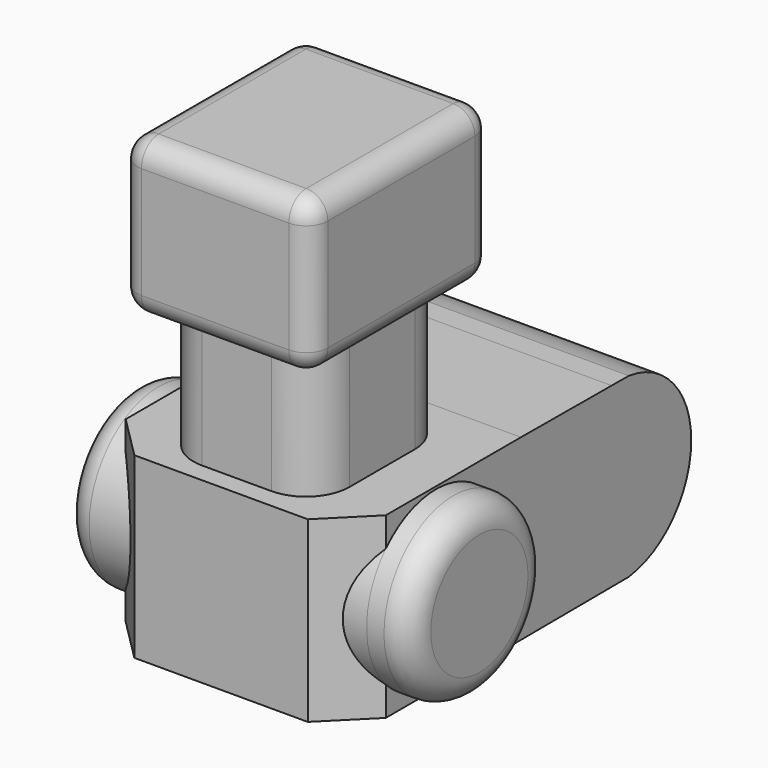
from build123d import *

# Parameters (mm, degrees)
F0_W          = 194.5625826716
F0_H          = 54.5296296477
F1_DEPTH      = 90
F0_W_2        = 261.9621157646
F0_H_2        = 41.3846671581
F0_H_3        = 48.0061769485
F2_DEPTH      = 110
F3_DEPTH      = 150
F4_DEPTH      = 200
F5_T1_DEPTH   = 170
F5_T3_DEPTH   = 211.9621157646
F5_T5_DEPTH   = 128.7816882133
F5_S9_W       = 25
F5_S9_H       = 25
F5_T10_DEPTH  = 25
F5_S15_W      = 25
F5_S15_H      = 25
F5_T16_DEPTH  = 25
F5_S21_W      = 25
F5_S21_H      = 25
F5_T22_DEPTH  = 25
F5_S27_W      = 25
F5_S27_H      = 25
F5_T28_DEPTH  = 25
F5_S33_W      = 25
F5_S33_H      = 25
F5_T34_DEPTH  = 25
F5_S39_W      = 25
F5_S39_H      = 25
F5_T40_DEPTH  = 25
F5_S45_W      = 25
F5_S45_H      = 25
F5_T46_DEPTH  = 25
F5_S51_W      = 25
F5_S51_H      = 25
F5_T52_DEPTH  = 25
F5_T58_DEPTH  = 211.9621157646
F5_T64_DEPTH  = 211.9621157646
F5_T70_DEPTH  = 211.9621157646
F5_T77_DEPTH  = 211.9621157646
F5_T83_DEPTH  = 211.9621157646
F5_T89_DEPTH  = 211.9621157646
F5_T95_DEPTH  = 211.9621157646
F5_T101_DEPTH = 211.9621157646
F5_T108_DEPTH = 211.9621157646
F5_T114_DEPTH = 211.9621157646
F6_R          = 50
F8_T4_DEPTH   = 462.9335014381
F8_S5_R       = 100
F8_T6_DEPTH   = 236
F8_T10_DEPTH  = 462.9335014381
F8_S11_R      = 100
F8_T12_DEPTH  = 236


# Not quite as in the source:
# - a fillet or chamfer that OpenCascade refuses, or shapes differently, is made with other operations: its cross-section is extruded or revolved along the edge and cut away or added


with BuildPart() as f1:
    # F0 (on Right) → F1 (new body, symmetric)
    with BuildSketch(Plane.YZ):
        with Locations((-2.7187086642, 130.1474161446)):
            Rectangle(F0_W, F0_H)
        Polygon((-100, 210.3845775127), (-100, 157.4122309685), (94.5625826716, 157.4122309685), (94.5625826716, 209.366121575), align=None)
        Polygon((-100, 248.4584450722), (-100, 210.3845775127), (94.5625826716, 209.366121575), (94.5625826716, 248.4584450722), align=None)
    extrude(amount=F1_DEPTH, both=True)

    # F0 (on Right) → F2 (join, symmetric)
    with BuildSketch(Plane.YZ):
        Polygon((-130.9810578823, 248.4584450722), (-100, 248.4584450722), (94.5625826716, 248.4584450722), (130.9810578823, 248.4584450722), (130.9810578823, 296.4646220207), (-130.9810578823, 296.4646220207), align=None)
        with Locations((0, 317.1569555998)):
            Rectangle(F0_W_2, F0_H_2)
        with Locations((0, 361.8523776531)):
            Rectangle(F0_W_2, F0_H_3)
        with Locations((0, 406.5477997065)):
            Rectangle(F0_W_2, F0_H_2)
    extrude(amount=F2_DEPTH, both=True)

    # F0 (on Right) → F3 (join, symmetric)
    with BuildSketch(Plane.YZ):
        with BuildLine():
            ThreePointArc((100, 0), (0, -100), (-100, 0))
            Line((-100, 0), (-100, 102.8826013207))
            Line((-100, 102.8826013207), (-122.4384903908, 102.8826013207))
            Line((-122.4384903908, 102.8826013207), (-122.4384903908, -102.8826013207))
            Line((-122.4384903908, -102.8826013207), (122.4384903908, -102.8826013207))
            Line((122.4384903908, -102.8826013207), (122.4384903908, 102.8826013207))
            Line((122.4384903908, 102.8826013207), (94.5625826716, 102.8826013207))
            Line((94.5625826716, 102.8826013207), (94.5625826716, 32.525650777))
            ThreePointArc((94.5625826716, 32.525650777), (98.6312786776, 16.4885071009), (100, 0))
        make_face()
        with BuildLine():
            Line((253.218506448, 102.1980211612), (122.4384903908, 102.8826013207))
            Line((122.4384903908, 102.8826013207), (122.4384903908, -102.8826013207))
            Line((122.4384903908, -102.8826013207), (253.218506448, -102.1980211612))
            ThreePointArc((253.218506448, -102.1980211612), (162.1847078204, 0), (253.218506448, 102.1980211612))
        make_face()
        with BuildLine():
            Line((277.9853632955, 102.0683767451), (253.218506448, 102.1980211612))
            ThreePointArc((253.218506448, 102.1980211612), (162.1847078204, 0), (253.218506448, -102.1980211612))
            Line((253.218506448, -102.1980211612), (277.9853632955, -102.0683767451))
            Line((277.9853632955, -102.0683767451), (277.9853632955, 102.0683767451))
        make_face()
        with BuildLine():
            ThreePointArc((367.9499104619, 0), (342.2485007293, 68.0286213263), (277.9853632955, 102.0683767451))
            Line((277.9853632955, 102.0683767451), (277.9853632955, -102.0683767451))
            ThreePointArc((277.9853632955, -102.0683767451), (342.2485007293, -68.0286213263), (367.9499104619, 0))
        make_face()
        with BuildLine():
            Line((-100, 102.8826013207), (-100, 0))
            ThreePointArc((-100, 0), (-16.4885071009, 98.6312786776), (94.5625826716, 32.525650777))
            Line((94.5625826716, 32.525650777), (94.5625826716, 102.8826013207))
            Line((94.5625826716, 102.8826013207), (-100, 102.8826013207))
        make_face()
    extrude(amount=F3_DEPTH, both=True)

    # F0 (on Right) → F4 (join, symmetric)
    with BuildSketch(Plane.YZ):
        with BuildLine():
            ThreePointArc((94.5625826716, 32.525650777), (-16.4885071009, 98.6312786776), (-100, 0))
            Line((-100, 0), (94.5625826716, 0))
            Line((94.5625826716, 0), (94.5625826716, 32.525650777))
        make_face()
        with BuildLine():
            Line((94.5625826716, 0), (-100, 0))
            ThreePointArc((-100, 0), (0, -100), (100, 0))
            ThreePointArc((100, 0), (98.6312786776, 16.4885071009), (94.5625826716, 32.525650777))
            Line((94.5625826716, 32.525650777), (94.5625826716, 0))
        make_face()
    extrude(amount=F4_DEPTH, both=True)

    # F5: fillet of radius 25 on 12 edges, made by hand

    # F5_s2 → F5_t1 (cut)
    with BuildSketch(Plane.YZ.offset(-85)):
        with BuildLine():
            ThreePointArc((-130.9810578823, 402.2401332855), (-123.658727412, 419.9178028152), (-105.9810578823, 427.2401332855))
            Line((-105.9810578823, 427.2401332855), (-130.9810578823, 427.2401332855))
            Line((-130.9810578823, 427.2401332855), (-130.9810578823, 402.2401332855))
        make_face()
        with BuildLine():
            ThreePointArc((130.9810578823, 402.2401332855), (123.658727412, 419.9178028152), (105.9810578823, 427.2401332855))
            Line((105.9810578823, 427.2401332855), (130.9810578823, 427.2401332855))
            Line((130.9810578823, 427.2401332855), (130.9810578823, 402.2401332855))
        make_face()
        with BuildLine():
            ThreePointArc((-105.9810578823, 248.4584450722), (-123.658727412, 255.7807755425), (-130.9810578823, 273.4584450722))
            Line((-130.9810578823, 273.4584450722), (-130.9810578823, 248.4584450722))
            Line((-130.9810578823, 248.4584450722), (-105.9810578823, 248.4584450722))
        make_face()
        with BuildLine():
            ThreePointArc((105.9810578823, 248.4584450722), (123.658727412, 255.7807755425), (130.9810578823, 273.4584450722))
            Line((130.9810578823, 273.4584450722), (130.9810578823, 248.4584450722))
            Line((130.9810578823, 248.4584450722), (105.9810578823, 248.4584450722))
        make_face()
    extrude(amount=F5_T1_DEPTH, mode=Mode.SUBTRACT)

    # F5_s4 → F5_t3 (cut)
    with BuildSketch(Plane.XZ.offset(-105.9810578823)):
        with BuildLine():
            ThreePointArc((110, 402.2401332855), (102.6776695297, 419.9178028152), (85, 427.2401332855))
            Line((85, 427.2401332855), (110, 427.2401332855))
            Line((110, 427.2401332855), (110, 402.2401332855))
        make_face()
        with BuildLine():
            ThreePointArc((-110, 402.2401332855), (-102.6776695297, 419.9178028152), (-85, 427.2401332855))
            Line((-85, 427.2401332855), (-110, 427.2401332855))
            Line((-110, 427.2401332855), (-110, 402.2401332855))
        make_face()
    extrude(amount=F5_T3_DEPTH, mode=Mode.SUBTRACT)

    # F5_s6 → F5_t5 (cut)
    with BuildSketch(Plane.XY.offset(273.4584450722)):
        with BuildLine():
            ThreePointArc((85, -130.9810578823), (102.6776695297, -123.658727412), (110, -105.9810578823))
            Line((110, -105.9810578823), (110, -130.9810578823))
            Line((110, -130.9810578823), (85, -130.9810578823))
        make_face()
        with BuildLine():
            ThreePointArc((85, 130.9810578823), (102.6776695297, 123.658727412), (110, 105.9810578823))
            Line((110, 105.9810578823), (110, 130.9810578823))
            Line((110, 130.9810578823), (85, 130.9810578823))
        make_face()
        with BuildLine():
            ThreePointArc((-110, -105.9810578823), (-102.6776695297, -123.658727412), (-85, -130.9810578823))
            Line((-85, -130.9810578823), (-110, -130.9810578823))
            Line((-110, -130.9810578823), (-110, -105.9810578823))
        make_face()
        with BuildLine():
            ThreePointArc((-110, 105.9810578823), (-102.6776695297, 123.658727412), (-85, 130.9810578823))
            Line((-85, 130.9810578823), (-110, 130.9810578823))
            Line((-110, 130.9810578823), (-110, 105.9810578823))
        make_face()
    extrude(amount=F5_T5_DEPTH, mode=Mode.SUBTRACT)


with BuildPart() as f5_tool8:
    # F5_s9 → F5_t10 (new body)
    with BuildSketch(Plane.XZ.offset(105.9810578823)):
        with Locations((97.5, 414.7401332855)):
            Rectangle(F5_S9_W, F5_S9_H)
    extrude(amount=F5_T10_DEPTH)

    # F5_s11 → F5_t12 (revolve, cut)
    with BuildSketch(Plane(origin=(85, -105.9810578823, 402.2401332855), x_dir=(-0.7071067812, 0, -0.7071067812), z_dir=(-0.7071067812, 0, 0.7071067812))):
        with BuildLine():
            ThreePointArc((0, -25), (25, 0), (0, 25))
            Line((0, 25), (0, -25))
        make_face()
    revolve(axis=Axis((85, -105.9810578823, 402.2401332855), (0, -1, 0)), mode=Mode.SUBTRACT)


with BuildPart() as f1_1:
    add(f1.part)

    # F5_t7: cut F5_tool8
    add(f5_tool8.part, mode=Mode.SUBTRACT)


with BuildPart() as f5_tool14:
    # F5_s15 → F5_t16 (new body)
    with BuildSketch(Plane.YZ.offset(-85)):
        with Locations((-118.4810578823, 414.7401332855)):
            Rectangle(F5_S15_W, F5_S15_H)
    extrude(amount=-F5_T16_DEPTH)

    # F5_s17 → F5_t18 (revolve, cut)
    with BuildSketch(Plane(origin=(-85, -105.9810578823, 402.2401332855), x_dir=(0, 0.7071067812, -0.7071067812), z_dir=(0, 0.7071067812, 0.7071067812))):
        with BuildLine():
            ThreePointArc((0, -25), (25, 0), (0, 25))
            Line((0, 25), (0, -25))
        make_face()
    revolve(axis=Axis((-85, -105.9810578823, 402.2401332855), (-1, 0, 0)), mode=Mode.SUBTRACT)


with BuildPart() as f1_2:
    add(f1_1.part)

    # F5_t13: cut F5_tool14
    add(f5_tool14.part, mode=Mode.SUBTRACT)


with BuildPart() as f5_tool20:
    # F5_s21 → F5_t22 (new body)
    with BuildSketch(Plane.XZ.offset(-105.9810578823)):
        with Locations((97.5, 414.7401332855)):
            Rectangle(F5_S21_W, F5_S21_H)
    extrude(amount=-F5_T22_DEPTH)

    # F5_s23 → F5_t24 (revolve, cut)
    with BuildSketch(Plane(origin=(85, 105.9810578823, 402.2401332855), x_dir=(-0.7071067812, 0, -0.7071067812), z_dir=(0.7071067812, 0, -0.7071067812))):
        with BuildLine():
            ThreePointArc((0, -25), (25, 0), (0, 25))
            Line((0, 25), (0, -25))
        make_face()
    revolve(axis=Axis((85, 105.9810578823, 402.2401332855), (0, 1, 0)), mode=Mode.SUBTRACT)


with BuildPart() as f1_3:
    add(f1_2.part)

    # F5_t19: cut F5_tool20
    add(f5_tool20.part, mode=Mode.SUBTRACT)


with BuildPart() as f5_tool26:
    # F5_s27 → F5_t28 (new body)
    with BuildSketch(Plane.YZ.offset(-85)):
        with Locations((118.4810578823, 414.7401332855)):
            Rectangle(F5_S27_W, F5_S27_H)
    extrude(amount=-F5_T28_DEPTH)

    # F5_s29 → F5_t30 (revolve, cut)
    with BuildSketch(Plane(origin=(-85, 105.9810578823, 402.2401332855), x_dir=(0, -0.7071067812, -0.7071067812), z_dir=(0, 0.7071067812, -0.7071067812))):
        with BuildLine():
            ThreePointArc((0, -25), (25, 0), (0, 25))
            Line((0, 25), (0, -25))
        make_face()
    revolve(axis=Axis((-85, 105.9810578823, 402.2401332855), (-1, 0, 0)), mode=Mode.SUBTRACT)


with BuildPart() as f1_4:
    add(f1_3.part)

    # F5_t25: cut F5_tool26
    add(f5_tool26.part, mode=Mode.SUBTRACT)


with BuildPart() as f5_tool32:
    # F5_s33 → F5_t34 (new body)
    with BuildSketch(Plane.XZ.offset(105.9810578823)):
        with Locations((97.5, 260.9584450722)):
            Rectangle(F5_S33_W, F5_S33_H)
    extrude(amount=F5_T34_DEPTH)

    # F5_s35 → F5_t36 (revolve, cut)
    with BuildSketch(Plane(origin=(85, -105.9810578823, 273.4584450722), x_dir=(-0.7071067812, 0, 0.7071067812), z_dir=(0.7071067812, 0, 0.7071067812))):
        with BuildLine():
            ThreePointArc((0, -25), (25, 0), (0, 25))
            Line((0, 25), (0, -25))
        make_face()
    revolve(axis=Axis((85, -105.9810578823, 273.4584450722), (0, -1, 0)), mode=Mode.SUBTRACT)


with BuildPart() as f1_5:
    add(f1_4.part)

    # F5_t31: cut F5_tool32
    add(f5_tool32.part, mode=Mode.SUBTRACT)


with BuildPart() as f5_tool38:
    # F5_s39 → F5_t40 (new body)
    with BuildSketch(Plane.XZ.offset(-105.9810578823)):
        with Locations((97.5, 260.9584450722)):
            Rectangle(F5_S39_W, F5_S39_H)
    extrude(amount=-F5_T40_DEPTH)

    # F5_s41 → F5_t42 (revolve, cut)
    with BuildSketch(Plane(origin=(85, 105.9810578823, 273.4584450722), x_dir=(-0.7071067812, 0, 0.7071067812), z_dir=(-0.7071067812, 0, -0.7071067812))):
        with BuildLine():
            ThreePointArc((0, -25), (25, 0), (0, 25))
            Line((0, 25), (0, -25))
        make_face()
    revolve(axis=Axis((85, 105.9810578823, 273.4584450722), (0, 1, 0)), mode=Mode.SUBTRACT)


with BuildPart() as f1_6:
    add(f1_5.part)

    # F5_t37: cut F5_tool38
    add(f5_tool38.part, mode=Mode.SUBTRACT)


with BuildPart() as f5_tool44:
    # F5_s45 → F5_t46 (new body)
    with BuildSketch(Plane.YZ.offset(-85)):
        with Locations((-118.4810578823, 260.9584450722)):
            Rectangle(F5_S45_W, F5_S45_H)
    extrude(amount=-F5_T46_DEPTH)

    # F5_s47 → F5_t48 (revolve, cut)
    with BuildSketch(Plane(origin=(-85, -105.9810578823, 273.4584450722), x_dir=(0, 0.7071067812, 0.7071067812), z_dir=(0, -0.7071067812, 0.7071067812))):
        with BuildLine():
            ThreePointArc((0, -25), (25, 0), (0, 25))
            Line((0, 25), (0, -25))
        make_face()
    revolve(axis=Axis((-85, -105.9810578823, 273.4584450722), (-1, 0, 0)), mode=Mode.SUBTRACT)


with BuildPart() as f1_7:
    add(f1_6.part)

    # F5_t43: cut F5_tool44
    add(f5_tool44.part, mode=Mode.SUBTRACT)


with BuildPart() as f5_tool50:
    # F5_s51 → F5_t52 (new body)
    with BuildSketch(Plane.YZ.offset(-85)):
        with Locations((118.4810578823, 260.9584450722)):
            Rectangle(F5_S51_W, F5_S51_H)
    extrude(amount=-F5_T52_DEPTH)

    # F5_s53 → F5_t54 (revolve, cut)
    with BuildSketch(Plane(origin=(-85, 105.9810578823, 273.4584450722), x_dir=(0, -0.7071067812, 0.7071067812), z_dir=(0, -0.7071067812, -0.7071067812))):
        with BuildLine():
            ThreePointArc((0, -25), (25, 0), (0, 25))
            Line((0, 25), (0, -25))
        make_face()
    revolve(axis=Axis((-85, 105.9810578823, 273.4584450722), (-1, 0, 0)), mode=Mode.SUBTRACT)


with BuildPart() as f1_8:
    add(f1_7.part)

    # F5_t49: cut F5_tool50
    add(f5_tool50.part, mode=Mode.SUBTRACT)


with BuildPart() as f5_tool56:
    # F5_s57 → F5_t58 (new body)
    with BuildSketch(Plane.XZ.offset(105.9810578823)):
        with BuildLine():
            ThreePointArc((85, 248.4584450722), (102.6776695297, 255.7807755425), (110, 273.4584450722))
            Line((110, 273.4584450722), (110, 248.4584450722))
            Line((110, 248.4584450722), (85, 248.4584450722))
        make_face()
    extrude(amount=-F5_T58_DEPTH)

    split(bisect_by=Plane.YZ.offset(90), keep=Keep.BOTTOM)

    split(bisect_by=Plane.XZ.offset(100), keep=Keep.TOP)


with BuildPart() as f1_9:
    add(f1_8.part)

    # F5_t55: cut F5_tool56
    add(f5_tool56.part, mode=Mode.SUBTRACT)


with BuildPart() as f5_tool62:
    # F5_s63 → F5_t64 (new body)
    with BuildSketch(Plane.XZ.offset(105.9810578823)):
        with BuildLine():
            ThreePointArc((85, 248.4584450722), (102.6776695297, 255.7807755425), (110, 273.4584450722))
            Line((110, 273.4584450722), (110, 248.4584450722))
            Line((110, 248.4584450722), (85, 248.4584450722))
        make_face()
    extrude(amount=-F5_T64_DEPTH)

    split(bisect_by=Plane.YZ.offset(90), keep=Keep.TOP)

    split(bisect_by=Plane.XZ.offset(100), keep=Keep.TOP)


with BuildPart() as f1_10:
    add(f1_9.part)

    # F5_t61: cut F5_tool62
    add(f5_tool62.part, mode=Mode.SUBTRACT)


with BuildPart() as f5_tool68:
    # F5_s69 → F5_t70 (new body)
    with BuildSketch(Plane.XZ.offset(105.9810578823)):
        with BuildLine():
            ThreePointArc((85, 248.4584450722), (102.6776695297, 255.7807755425), (110, 273.4584450722))
            Line((110, 273.4584450722), (110, 248.4584450722))
            Line((110, 248.4584450722), (85, 248.4584450722))
        make_face()
    extrude(amount=-F5_T70_DEPTH)

    split(bisect_by=Plane.YZ.offset(90), keep=Keep.TOP)

    split(bisect_by=Plane.XZ.offset(-94.5625826716), keep=Keep.TOP)

    split(bisect_by=Plane.XZ.offset(100), keep=Keep.BOTTOM)


with BuildPart() as f1_11:
    add(f1_10.part)

    # F5_t67: cut F5_tool68
    add(f5_tool68.part, mode=Mode.SUBTRACT)


with BuildPart() as f5_tool75:
    # F5_s76 → F5_t77 (new body)
    with BuildSketch(Plane.XZ.offset(105.9810578823)):
        with BuildLine():
            ThreePointArc((85, 248.4584450722), (102.6776695297, 255.7807755425), (110, 273.4584450722))
            Line((110, 273.4584450722), (110, 248.4584450722))
            Line((110, 248.4584450722), (85, 248.4584450722))
        make_face()
    extrude(amount=-F5_T77_DEPTH)

    split(bisect_by=Plane.YZ.offset(90), keep=Keep.BOTTOM)

    split(bisect_by=Plane.XZ.offset(-94.5625826716), keep=Keep.BOTTOM)


with BuildPart() as f1_12:
    add(f1_11.part)

    # F5_t74: cut F5_tool75
    add(f5_tool75.part, mode=Mode.SUBTRACT)


with BuildPart() as f5_tool81:
    # F5_s82 → F5_t83 (new body)
    with BuildSketch(Plane.XZ.offset(105.9810578823)):
        with BuildLine():
            ThreePointArc((85, 248.4584450722), (102.6776695297, 255.7807755425), (110, 273.4584450722))
            Line((110, 273.4584450722), (110, 248.4584450722))
            Line((110, 248.4584450722), (85, 248.4584450722))
        make_face()
    extrude(amount=-F5_T83_DEPTH)

    split(bisect_by=Plane.YZ.offset(90), keep=Keep.TOP)

    split(bisect_by=Plane.XZ.offset(-94.5625826716), keep=Keep.BOTTOM)


with BuildPart() as f1_13:
    add(f1_12.part)

    # F5_t80: cut F5_tool81
    add(f5_tool81.part, mode=Mode.SUBTRACT)


with BuildPart() as f5_tool87:
    # F5_s88 → F5_t89 (new body)
    with BuildSketch(Plane.XZ.offset(105.9810578823)):
        with BuildLine():
            ThreePointArc((-85, 248.4584450722), (-102.6776695297, 255.7807755425), (-110, 273.4584450722))
            Line((-110, 273.4584450722), (-110, 248.4584450722))
            Line((-110, 248.4584450722), (-85, 248.4584450722))
        make_face()
    extrude(amount=-F5_T89_DEPTH)

    split(bisect_by=Plane.YZ.offset(-90), keep=Keep.TOP)

    split(bisect_by=Plane.XZ.offset(100), keep=Keep.TOP)


with BuildPart() as f1_14:
    add(f1_13.part)

    # F5_t86: cut F5_tool87
    add(f5_tool87.part, mode=Mode.SUBTRACT)


with BuildPart() as f5_tool93:
    # F5_s94 → F5_t95 (new body)
    with BuildSketch(Plane.XZ.offset(105.9810578823)):
        with BuildLine():
            ThreePointArc((-85, 248.4584450722), (-102.6776695297, 255.7807755425), (-110, 273.4584450722))
            Line((-110, 273.4584450722), (-110, 248.4584450722))
            Line((-110, 248.4584450722), (-85, 248.4584450722))
        make_face()
    extrude(amount=-F5_T95_DEPTH)

    split(bisect_by=Plane.YZ.offset(-90), keep=Keep.BOTTOM)

    split(bisect_by=Plane.XZ.offset(100), keep=Keep.TOP)


with BuildPart() as f1_15:
    add(f1_14.part)

    # F5_t92: cut F5_tool93
    add(f5_tool93.part, mode=Mode.SUBTRACT)


with BuildPart() as f5_tool99:
    # F5_s100 → F5_t101 (new body)
    with BuildSketch(Plane.XZ.offset(105.9810578823)):
        with BuildLine():
            ThreePointArc((-85, 248.4584450722), (-102.6776695297, 255.7807755425), (-110, 273.4584450722))
            Line((-110, 273.4584450722), (-110, 248.4584450722))
            Line((-110, 248.4584450722), (-85, 248.4584450722))
        make_face()
    extrude(amount=-F5_T101_DEPTH)

    split(bisect_by=Plane.XZ.offset(-94.5625826716), keep=Keep.TOP)

    split(bisect_by=Plane.YZ.offset(-90), keep=Keep.BOTTOM)

    split(bisect_by=Plane.XZ.offset(100), keep=Keep.BOTTOM)


with BuildPart() as f1_16:
    add(f1_15.part)

    # F5_t98: cut F5_tool99
    add(f5_tool99.part, mode=Mode.SUBTRACT)


with BuildPart() as f5_tool106:
    # F5_s107 → F5_t108 (new body)
    with BuildSketch(Plane.XZ.offset(105.9810578823)):
        with BuildLine():
            ThreePointArc((-85, 248.4584450722), (-102.6776695297, 255.7807755425), (-110, 273.4584450722))
            Line((-110, 273.4584450722), (-110, 248.4584450722))
            Line((-110, 248.4584450722), (-85, 248.4584450722))
        make_face()
    extrude(amount=-F5_T108_DEPTH)

    split(bisect_by=Plane.XZ.offset(-94.5625826716), keep=Keep.BOTTOM)

    split(bisect_by=Plane.YZ.offset(-90), keep=Keep.TOP)


with BuildPart() as f1_17:
    add(f1_16.part)

    # F5_t105: cut F5_tool106
    add(f5_tool106.part, mode=Mode.SUBTRACT)


with BuildPart() as f5_tool112:
    # F5_s113 → F5_t114 (new body)
    with BuildSketch(Plane.XZ.offset(105.9810578823)):
        with BuildLine():
            ThreePointArc((-85, 248.4584450722), (-102.6776695297, 255.7807755425), (-110, 273.4584450722))
            Line((-110, 273.4584450722), (-110, 248.4584450722))
            Line((-110, 248.4584450722), (-85, 248.4584450722))
        make_face()
    extrude(amount=-F5_T114_DEPTH)

    split(bisect_by=Plane.XZ.offset(-94.5625826716), keep=Keep.BOTTOM)

    split(bisect_by=Plane.YZ.offset(-90), keep=Keep.BOTTOM)


with BuildPart() as f1_18:
    add(f1_17.part)

    # F5_t111: cut F5_tool112
    add(f5_tool112.part, mode=Mode.SUBTRACT)

    # F6
    f6_edges = [f1_18.edges().sort_by_distance(p)[0] for p in [
        (90, -100, 175.923074),
        (90, 94.562583, 175.923074),
        (-90, 94.562583, 175.923074),
        (-90, -100, 175.923074),
    ]]
    fillet(f6_edges, radius=F6_R)

    # F7: fillet of radius 30 on 2 edges, made by hand

    # F7_s1 → F7_t2 (revolve, cut)
    with BuildSketch(Plane.XY):
        with BuildLine():
            ThreePointArc((170, -100), (191.2132034356, -91.2132034356), (200, -70))
            Line((200, -70), (200, -100))
            Line((200, -100), (170, -100))
        make_face()
    revolve(axis=Axis((200, 0, 0), (1, 0, 0)), mode=Mode.SUBTRACT)

    # F7_s3 → F7_t4 (revolve, cut)
    with BuildSketch(Plane.XY):
        with BuildLine():
            ThreePointArc((-170, -100), (-191.2132034356, -91.2132034356), (-200, -70))
            Line((-200, -70), (-200, -100))
            Line((-200, -100), (-170, -100))
        make_face()
    revolve(axis=Axis((-200, 0, 0), (1, 0, 0)), mode=Mode.SUBTRACT)

    # F8: chamfer of 50 on 2 edges, made by hand


with BuildPart() as f8_tool2:
    # F8_s3 → F8_t4 (new body)
    with BuildSketch(Plane.XY.offset(231.466750719)):
        Polygon((-150, -72.4384903908), (-100, -122.4384903908), (-150, -122.4384903908), align=None)
    extrude(amount=-F8_T4_DEPTH)

    # F8_s5 → F8_t6 (cut, symmetric)
    with BuildSketch(Plane.YZ.offset(-125)):
        Circle(F8_S5_R)
    extrude(amount=F8_T6_DEPTH, both=True, mode=Mode.SUBTRACT)


with BuildPart() as f1_19:
    add(f1_18.part)

    # F8_t1: cut F8_tool2
    add(f8_tool2.part, mode=Mode.SUBTRACT)


with BuildPart() as f8_tool8:
    # F8_s9 → F8_t10 (new body)
    with BuildSketch(Plane.XY.offset(231.466750719)):
        Polygon((100, -122.4384903908), (150, -72.4384903908), (150, -122.4384903908), align=None)
    extrude(amount=-F8_T10_DEPTH)

    # F8_s11 → F8_t12 (cut, symmetric)
    with BuildSketch(Plane.YZ.offset(125)):
        Circle(F8_S11_R)
    extrude(amount=F8_T12_DEPTH, both=True, mode=Mode.SUBTRACT)


with BuildPart() as f1_20:
    add(f1_19.part)

    # F8_t7: cut F8_tool8
    add(f8_tool8.part, mode=Mode.SUBTRACT)


solid = f1_20.part
